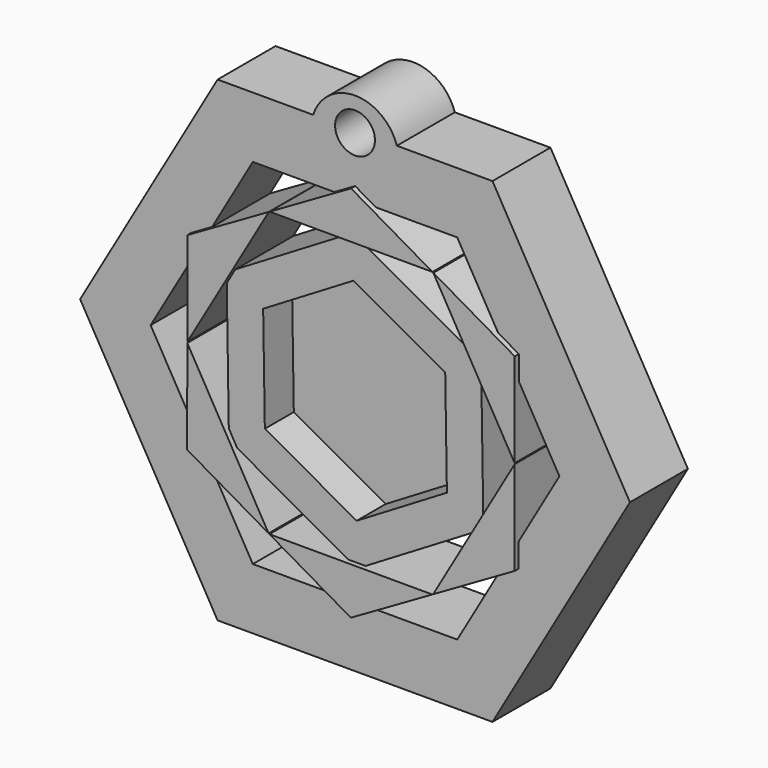
from build123d import *

# Parameters (mm, degrees)
F1_DEPTH  = 5.08
F2_R      = 3.0783155003
F3_DEPTH  = 5.08
F5_D      = 2.794
F7_DEPTH  = 5.08
F8_SCALE  = 1.07
F10_DEPTH = 5.08
F11_DEPTH = 1.4986
F14_T     = -2.54


with BuildPart() as f1:
    # F0 (on Front) → F1 (new body)
    with BuildSketch(Plane.XZ):
        Polygon((-9.6395150281, -16.6961297889), (9.6395150281, -16.6961297889), (19.2790300561, 0), (9.6395150281, 16.6961297889), (-9.6395150281, 16.6961297889), (-19.2790300561, 0), align=None)
        Polygon((14.3360053558, 0), (7.1680026779, -12.4153448269), (-7.1680026779, -12.4153448269), (-14.3360053558, 0), (-7.1680026779, 12.4153448269), (7.1680026779, 12.4153448269), align=None, mode=Mode.SUBTRACT)
    extrude(amount=F1_DEPTH)

    # F2 (on Front) → F3 (join)
    with BuildSketch(Plane.XZ):
        with Locations((0, 15.7666336745)):
            Circle(F2_R)
    extrude(amount=F3_DEPTH)

    # F5 (through all)
    with Locations(Plane(origin=(0, 0, 0), x_dir=(1, 0, 0), z_dir=(0, 1, 0))):
        with Locations((0, -16.5367200971)):
            Hole(F5_D / 2)


with BuildPart() as f7:
    # F6 (on face) → F7 (new body)
    with BuildSketch(Plane.XZ.offset(5.08)):
        Polygon((5.3438666064, 9.3036550664), (0.0089031178, 12.3889116569), (-5.3300339055, 9.3115884774), align=None)
    extrude(amount=-F7_DEPTH)


with BuildPart() as f7b:
    # F6 (on face) → F7, piece 2 (new body)
    with BuildSketch(Plane.XZ.offset(5.08)):
        Polygon((10.733563779, 6.1867455022), (5.3990552183, 9.2717390039), (10.7291349388, 0.0239032976), align=None)
    extrude(amount=-F7_DEPTH)


with BuildPart() as f7c:
    # F6 (on face) → F7, piece 3 (new body)
    with BuildSketch(Plane.XZ.offset(5.08)):
        Polygon((-10.7290891237, 0.0398494735), (-5.3852683323, 9.2797517688), (-10.7246606612, 6.2021661546), align=None)
    extrude(amount=-F7_DEPTH)


with BuildPart() as f7d:
    # F6 (on face) → F7, piece 4 (new body)
    with BuildSketch(Plane.XZ.offset(5.08)):
        Polygon((10.7246606612, -6.2021661546), (10.7290891237, -0.0398494735), (5.3852683323, -9.2797517688), align=None)
    extrude(amount=-F7_DEPTH)


with BuildPart() as f7e:
    # F6 (on face) → F7, piece 5 (new body)
    with BuildSketch(Plane.XZ.offset(5.08)):
        Polygon((-5.3990552183, -9.2717390039), (-10.7291349388, -0.0239032976), (-10.733563779, -6.1867455022), align=None)
    extrude(amount=-F7_DEPTH)


with BuildPart() as f7f:
    # F6 (on face) → F7, piece 6 (new body)
    with BuildSketch(Plane.XZ.offset(5.08)):
        Polygon((-0.0089031178, -12.3889116569), (5.3300339055, -9.3115884774), (-5.3438666064, -9.3036550664), align=None)
    extrude(amount=-F7_DEPTH)


with BuildPart() as f7g:
    # F6 (on face) → F7, piece 7 (new body)
    with BuildSketch(Plane.XZ.offset(5.08)):
        Polygon((8.0364226741, -4.6477983427), (8.0398727238, -0.0059756613), (4.025102565, -6.9597615571), align=None)
    extrude(amount=-F7_DEPTH)


with BuildPart() as f7b_1:
    # F8: moved
    add(f7b.part.scale(F8_SCALE))


with BuildPart() as f7d_1:
    # F8: moved
    add(f7d.part.scale(F8_SCALE))


with BuildPart() as f7f_1:
    # F8: moved
    add(f7f.part.scale(F8_SCALE))


with BuildPart() as f7e_1:
    # F8: moved
    add(f7e.part.scale(F8_SCALE))


with BuildPart() as f7c_1:
    # F8: moved
    add(f7c.part.scale(F8_SCALE))


with BuildPart() as f7_1:
    # F8: moved
    add(f7.part.scale(F8_SCALE))


with BuildPart() as f10:
    # F9 (on face) → F10 (new body)
    with BuildSketch(Plane.XZ.offset(5.08)):
        Polygon((0.1654340336, -10.3049334588), (9.0070511764, -5.0091966537), (8.8416171429, 5.2957368051), (-0.1654340336, 10.3049334588), (-9.0070511764, 5.0091966537), (-8.8416171429, -5.2957368051), align=None)
    extrude(amount=-F10_DEPTH)

    # F14
    f14_openings = [f10.faces().sort_by_distance(p)[0] for p in [
        (0, -5.08, 0),
    ]]
    offset(amount=F14_T, openings=f14_openings)


with BuildPart() as f11:
    # F11 (new): a face of the model
    f11_faces = [f7g.part.faces().sort_by_distance(p)[0] for p in [
        (6.7004659876, -5.08, -3.8711785204),
    ]]
    extrude(f11_faces, amount=-F11_DEPTH)


solid = Compound([f1.part, f7b_1.part, f7d_1.part, f7f_1.part, f7e_1.part, f7c_1.part, f7_1.part, f10.part])
